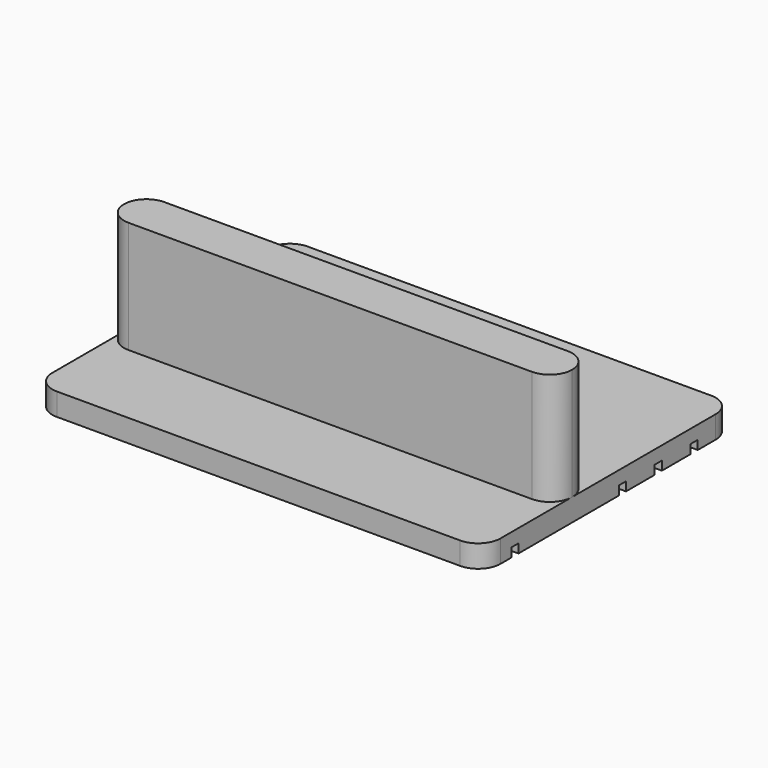
from build123d import *

# Parameters (mm, degrees)
F0_W           = 50
F0_H           = 5
F0_H_2         = 4
F0_H_3         = 1
F1_DEPTH       = 2.5
F2_DEPTH       = 15
F3_R           = 2.49999
F4_D           = 3.2
F4_DEPTH       = 12
F4_CSINK_D     = 8.96
F4_CSINK_ANGLE = 90
F4_TIP         = 0.9613769904
F5_DEPTH       = 1


# Not quite as in the source:
# - a fillet or chamfer is up to 0.001 mm smaller than in the source, because OpenCascade refuses the exact size


with BuildPart() as f1:
    # F0 (on Top) → F1 (new body)
    with BuildSketch(Plane.XY):
        with Locations((0, 15)):
            Rectangle(F0_W, F0_H)
        with Locations((0, -5.5)):
            Rectangle(F0_W, F0_H_2)
        with Locations((0, -15.5)):
            Rectangle(F0_W, F0_H_2)
        with Locations((0, -13)):
            Rectangle(F0_W, F0_H_3)
        with Locations((0, -10.5)):
            Rectangle(F0_W, F0_H_2)
        with Locations((0, -3)):
            Rectangle(F0_W, F0_H_3)
        with Locations((0, -0.5)):
            Rectangle(F0_W, F0_H_2)
        with Locations((0, 7)):
            Rectangle(F0_W, F0_H_3)
        with Locations((0, 9.5)):
            Rectangle(F0_W, F0_H_2)
        with Locations((0, 12)):
            Rectangle(F0_W, F0_H_3)
        with Locations((0, -8)):
            Rectangle(F0_W, F0_H_3)
        with Locations((0, 2)):
            Rectangle(F0_W, F0_H_3)
        with Locations((0, 4.5)):
            Rectangle(F0_W, F0_H_2)
    extrude(amount=F1_DEPTH)

    # F0 (on Top) → F2 (join)
    with BuildSketch(Plane.XY):
        with Locations((0, -5.5)):
            Rectangle(F0_W, F0_H_2)
        with Locations((0, -3)):
            Rectangle(F0_W, F0_H_3)
    extrude(amount=F2_DEPTH)

    # F3 (radius 2.5 in the source; OpenCascade refuses exactly that, so slightly less here)
    f3_edges = [f1.edges().sort_by_distance(p)[0] for p in [
        (-25, 17.5, 1.25),
        (25, 17.5, 1.25),
        (25, -2.5, 8.75),
        (25, -7.5, 8.75),
        (-25, -2.5, 8.75),
        (-25, -7.5, 8.75),
        (-25, -17.5, 1.25),
        (25, -17.5, 1.25),
    ]]
    fillet(f3_edges, radius=F3_R)

    # F4
    with Locations(Plane(origin=(0, 0, 0), x_dir=(1, 0, 0), z_dir=(0, 0, -1))):
        with Locations((20, 5), (10, 5), (0, 5), (-10, 5), (-20, 5)):
            CounterSinkHole(F4_D / 2, F4_CSINK_D / 2, depth=F4_DEPTH, counter_sink_angle=F4_CSINK_ANGLE)
            with Locations((0, 0, -(F4_DEPTH + F4_TIP / 2))):  # 118° drill point
                Cone(0, F4_D / 2, F4_TIP, mode=Mode.SUBTRACT)

    # F0 (on Top) → F5 (cut)
    with BuildSketch(Plane.XY):
        with Locations((0, -13)):
            Rectangle(F0_W, F0_H_3)
        with Locations((0, 2)):
            Rectangle(F0_W, F0_H_3)
        with Locations((0, 7)):
            Rectangle(F0_W, F0_H_3)
        with Locations((0, 12)):
            Rectangle(F0_W, F0_H_3)
    extrude(amount=F5_DEPTH, mode=Mode.SUBTRACT)


solid = f1.part
